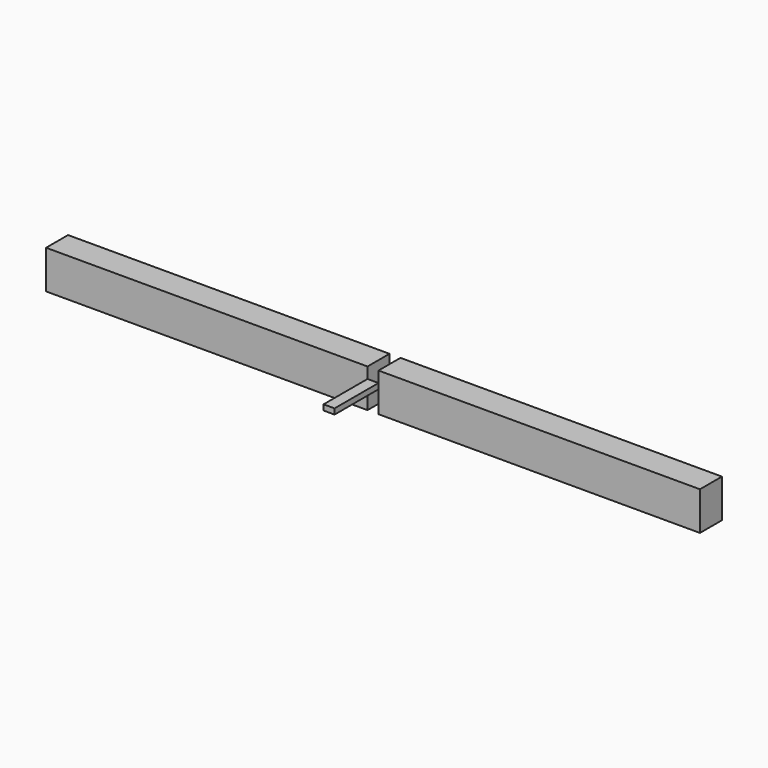
from build123d import *

# Parameters (mm, degrees)
F1_DEPTH = 59.5
F0_W     = 10
F0_H     = 1
F2_DEPTH = 1
F3_W     = 25.6279632449
F3_H     = 26.6232225113
F4_DEPTH = 1


# Not quite as in the source:
# - a feature of the source that left no trace in its solid (it failed there, or was rolled back) is left out


with BuildPart() as f1:
    # F0 (on Right) → F1 (new body, symmetric)
    with BuildSketch(Plane.YZ):
        Polygon((-20, -3), (-25, -3), (-25, -5), (-25, -6), (-25, -10), (-20, -10), align=None)
    extrude(amount=F1_DEPTH, both=True)

    # F3 (on Right) → F4 (cut, symmetric)
    with BuildSketch(Plane.YZ):
        with Locations((-24.7571095824, -6.4691940788)):
            Rectangle(F3_W, F3_H)
    extrude(amount=F4_DEPTH, both=True, mode=Mode.SUBTRACT)


with BuildPart() as f2:
    # F0 (on Right) → F2 (new body, symmetric)
    with BuildSketch(Plane.YZ):
        with Locations((-30, -5.5)):
            Rectangle(F0_W, F0_H)
    extrude(amount=F2_DEPTH, both=True)


solid = Compound([f1.part, f2.part])
